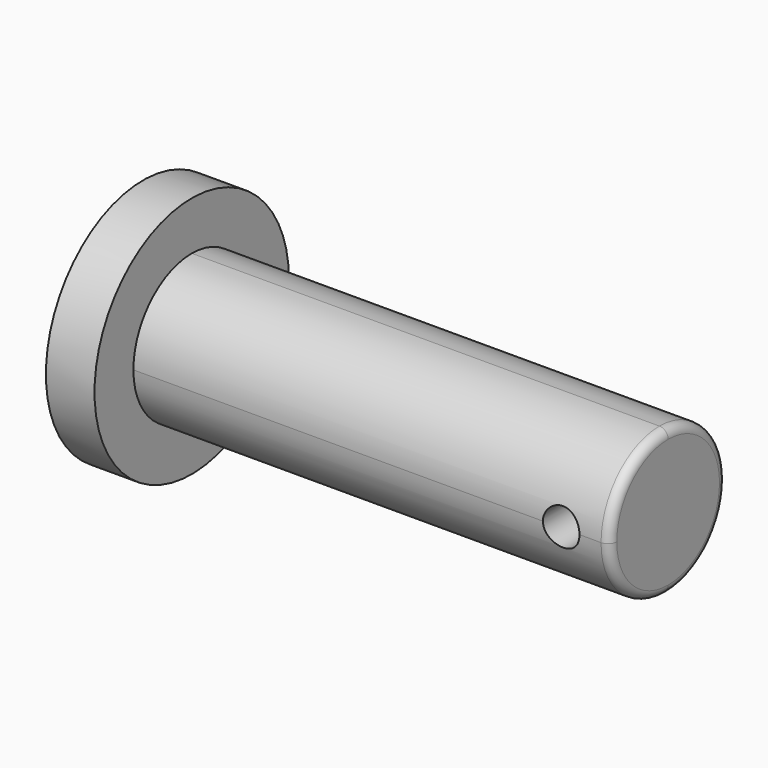
from build123d import *

# Parameters (mm, degrees)
F0_R        = 15.875
F1_DEPTH    = 6.35
F2_W        = 9.525
F2_H        = 9.525
F3_DEPTH    = 62.23
F4_R        = 2.3876
F5_DEPTH    = 25.4
F6_T1_DEPTH = 62.23
F7_R        = 1.143


# Not quite as in the source:
# - a fillet or chamfer that OpenCascade refuses, or shapes differently, is made with other operations: its cross-section is extruded or revolved along the edge and cut away or added


with BuildPart() as f1:
    # F0 (on Right) → F1 (new body)
    with BuildSketch(Plane.YZ):
        Circle(F0_R)
    extrude(amount=F1_DEPTH)

    # F2 (on face) → F3 (join)
    with BuildSketch(Plane.YZ.offset(6.35)):
        with Locations((4.7625, 4.7625)):
            Rectangle(F2_W, F2_H)
        with Locations((-4.7625, -4.7625)):
            Rectangle(F2_W, F2_H)
        with Locations((-4.7625, 4.7625)):
            Rectangle(F2_W, F2_H)
        with Locations((4.7625, -4.7625)):
            Rectangle(F2_W, F2_H)
    extrude(amount=F3_DEPTH)

    # F4 (on face) → F5 (cut)
    with BuildSketch(Plane.XZ.offset(9.525)):
        with Locations((62.23, 0)):
            Circle(F4_R)
    extrude(amount=-F5_DEPTH, mode=Mode.SUBTRACT)

    # F6: fillet of radius 9.525 on 4 edges, made by hand

    # F6_s2 → F6_t1 (cut)
    with BuildSketch(Plane.YZ.offset(6.35)):
        with BuildLine():
            ThreePointArc((0, 9.525), (-6.7351920908, 6.7351920908), (-9.525, 0))
            Line((-9.525, 0), (-9.7155, 0))
            Line((-9.7155, 0), (-9.7155, 9.7155))
            Line((-9.7155, 9.7155), (0, 9.7155))
            Line((0, 9.7155), (0, 9.525))
        make_face()
        with BuildLine():
            ThreePointArc((0, 9.525), (6.7351920908, 6.7351920908), (9.525, 0))
            Line((9.525, 0), (9.7155, 0))
            Line((9.7155, 0), (9.7155, 9.7155))
            Line((9.7155, 9.7155), (0, 9.7155))
            Line((0, 9.7155), (0, 9.525))
        make_face()
        with BuildLine():
            ThreePointArc((-9.525, 0), (-6.7351920908, -6.7351920908), (0, -9.525))
            Line((0, -9.525), (0, -9.7155))
            Line((0, -9.7155), (-9.7155, -9.7155))
            Line((-9.7155, -9.7155), (-9.7155, 0))
            Line((-9.7155, 0), (-9.525, 0))
        make_face()
        with BuildLine():
            ThreePointArc((0, -9.525), (6.7351920908, -6.7351920908), (9.525, 0))
            Line((9.525, 0), (9.7155, 0))
            Line((9.7155, 0), (9.7155, -9.7155))
            Line((9.7155, -9.7155), (0, -9.7155))
            Line((0, -9.7155), (0, -9.525))
        make_face()
    extrude(amount=F6_T1_DEPTH, mode=Mode.SUBTRACT)

    # F7
    f7_edges = [f1.edges().sort_by_distance(p)[0] for p in [
        (68.58, -6.735192, -6.735192),
    ]]
    fillet(f7_edges, radius=F7_R)


solid = f1.part
